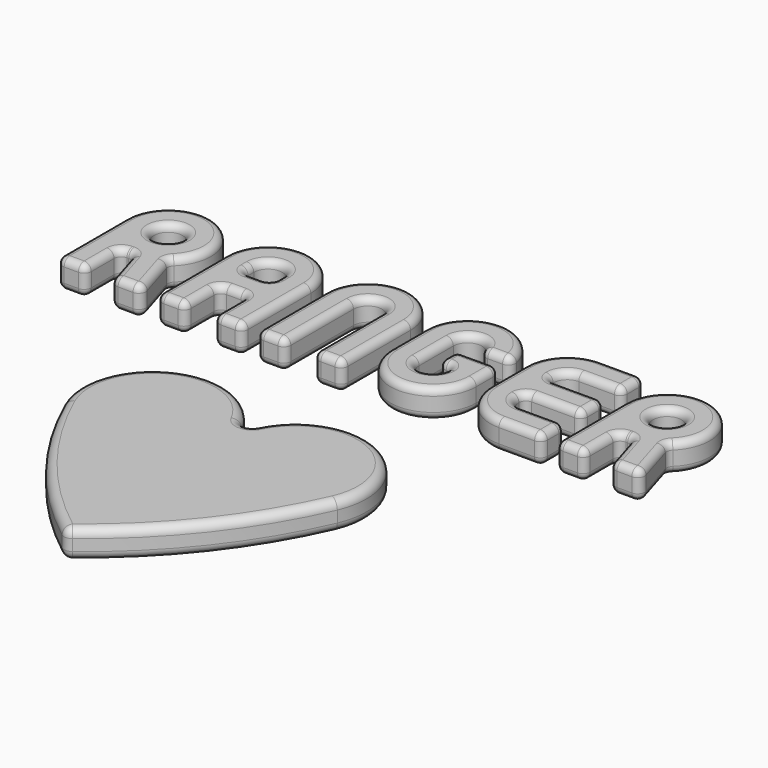
from build123d import *

# Parameters (mm, degrees)
F1_DEPTH = 1
F0_R     = 0.5
F2_R     = 0.24999
F2_2_R   = 0.24999
F2_3_R   = 0.24999
F2_4_R   = 0.24999
F2_5_R   = 0.24999
F2_6_R   = 0.24999
F4_DEPTH = 1
F5_R     = 0.3


# Not quite as in the source:
# - a fillet or chamfer is up to 0.001 mm smaller than in the source, because OpenCascade refuses the exact size


with BuildPart() as f1:
    # F0 (on Top) → F1 (new body)
    with BuildSketch(Plane.XY):
        with BuildLine():
            ThreePointArc((-12, 3), (-13.5, 4.5), (-15, 3))
            Line((-15, 3), (-15, 0))
            Line((-15, 0), (-14, 0))
            Line((-14, 0), (-14, 1.5))
            Line((-14, 1.5), (-13, 1.5))
            Line((-13, 1.5), (-13, 0))
            Line((-13, 0), (-12, 0))
            Line((-12, 0), (-12, 3))
        make_face()
        with BuildLine():
            ThreePointArc((-14, 3), (-13.5, 3.5), (-13, 3))
            Line((-13, 3), (-13, 2.5))
            Line((-13, 2.5), (-14, 2.5))
            Line((-14, 2.5), (-14, 3))
        make_face(mode=Mode.SUBTRACT)
    extrude(amount=F1_DEPTH)

    # F2#2 (radius 0.25 in the source; OpenCascade refuses exactly that, so slightly less here)
    f2_2_edges = [f1.edges().sort_by_distance(p)[0] for p in [
        (-13.5, 4.5, 1),
        (-15, 1.5, 1),
        (-14.5, 0, 1),
        (-14, 0.75, 1),
        (-13.5, 1.5, 1),
        (-13, 0.75, 1),
        (-12.5, 0, 1),
        (-12, 1.5, 1),
        (-13.5, 3.5, 1),
        (-13, 2.75, 1),
        (-13.5, 2.5, 1),
        (-14, 2.75, 1),
        (-13.5, 4.5, 0),
        (-15, 1.5, 0),
        (-14.5, 0, 0),
        (-14, 0.75, 0),
        (-13.5, 1.5, 0),
        (-13, 0.75, 0),
        (-12.5, 0, 0),
        (-12, 1.5, 0),
        (-13.5, 3.5, 0),
        (-13, 2.75, 0),
        (-13.5, 2.5, 0),
        (-14, 2.75, 0),
        (-13, 0, 0.5),
        (-12, 0, 0.5),
        (-13, 2.5, 0.5),
        (-14, 2.5, 0.5),
        (-14, 1.5, 0.5),
        (-13, 1.5, 0.5),
        (-15, 0, 0.5),
        (-14, 0, 0.5),
    ]]
    fillet(f2_2_edges, radius=F2_2_R)


with BuildPart() as f1b:
    # F0 (on Top) → F1, piece 2 (new body)
    with BuildSketch(Plane.XY):
        with BuildLine():
            ThreePointArc((-8.5, 3), (-10, 4.5), (-11.5, 3))
            Line((-11.5, 3), (-11.5, 0))
            Line((-11.5, 0), (-10.5, 0))
            Line((-10.5, 0), (-10.5, 3))
            ThreePointArc((-10.5, 3), (-10, 3.5), (-9.5, 3))
            Line((-9.5, 3), (-9.5, 0))
            Line((-9.5, 0), (-8.5, 0))
            Line((-8.5, 0), (-8.5, 3))
        make_face()
    extrude(amount=F1_DEPTH)

    # F2#3 (radius 0.25 in the source; OpenCascade refuses exactly that, so slightly less here)
    f2_3_edges = [f1b.edges().sort_by_distance(p)[0] for p in [
        (-10, 4.5, 1),
        (-11.5, 1.5, 1),
        (-11, 0, 1),
        (-10.5, 1.5, 1),
        (-10, 3.5, 1),
        (-9.5, 1.5, 1),
        (-9, 0, 1),
        (-8.5, 1.5, 1),
        (-10, 4.5, 0),
        (-11.5, 1.5, 0),
        (-11, 0, 0),
        (-10.5, 1.5, 0),
        (-10, 3.5, 0),
        (-9.5, 1.5, 0),
        (-9, 0, 0),
        (-8.5, 1.5, 0),
        (-9.5, 0, 0.5),
        (-8.5, 0, 0.5),
        (-11.5, 0, 0.5),
        (-10.5, 0, 0.5),
    ]]
    fillet(f2_3_edges, radius=F2_3_R)


with BuildPart() as f1c:
    # F0 (on Top) → F1, piece 3 (new body)
    with BuildSketch(Plane.XY):
        with BuildLine():
            Line((-7, 1.5), (-7, 3))
            ThreePointArc((-7, 3), (-6.5, 3.5), (-6, 3))
            Line((-6, 3), (-5, 3))
            ThreePointArc((-5, 3), (-6.5, 4.5), (-8, 3))
            Line((-8, 3), (-8, 1.5))
            ThreePointArc((-8, 1.5), (-6.5, 0), (-5, 1.5))
            Line((-5, 1.5), (-5, 2.5))
            Line((-5, 2.5), (-6.5, 2.5))
            Line((-6.5, 2.5), (-6.5, 1.75))
            Line((-6.5, 1.75), (-6, 1.75))
            Line((-6, 1.75), (-6, 1.5))
            ThreePointArc((-6, 1.5), (-6.5, 1), (-7, 1.5))
        make_face()
    extrude(amount=F1_DEPTH)

    # F2#4 (radius 0.25 in the source; OpenCascade refuses exactly that, so slightly less here)
    f2_4_edges = [f1c.edges().sort_by_distance(p)[0] for p in [
        (-6, 1.625, 1),
        (-6.5, 1, 1),
        (-7, 2.25, 1),
        (-6.5, 3.5, 1),
        (-5.5, 3, 1),
        (-6.5, 4.5, 1),
        (-8, 2.25, 1),
        (-6.5, 0, 1),
        (-5, 2, 1),
        (-5.75, 2.5, 1),
        (-6.5, 2.125, 1),
        (-6.25, 1.75, 1),
        (-6, 1.625, 0),
        (-6.5, 1, 0),
        (-7, 2.25, 0),
        (-6.5, 3.5, 0),
        (-5.5, 3, 0),
        (-6.5, 4.5, 0),
        (-8, 2.25, 0),
        (-6.5, 0, 0),
        (-5, 2, 0),
        (-5.75, 2.5, 0),
        (-6.5, 2.125, 0),
        (-6.25, 1.75, 0),
        (-5, 2.5, 0.5),
        (-6.5, 2.5, 0.5),
        (-6, 1.5, 0.5),
        (-7, 1.5, 0.5),
        (-8, 1.5, 0.5),
        (-5, 1.5, 0.5),
        (-6.5, 1.75, 0.5),
        (-6, 1.75, 0.5),
        (-6, 3, 0.5),
        (-5, 3, 0.5),
        (-7, 3, 0.5),
    ]]
    fillet(f2_4_edges, radius=F2_4_R)


with BuildPart() as f1d:
    # F0 (on Top) → F1, piece 4 (new body)
    with BuildSketch(Plane.XY):
        with BuildLine():
            ThreePointArc((-3, 4.5), (-4.0606601718, 4.0606601718), (-4.5, 3))
            Line((-4.5, 3), (-4.5, 1.5))
            ThreePointArc((-4.5, 1.5), (-4.0606601718, 0.4393398282), (-3, 0))
            Line((-3, 0), (-1.5, 0))
            Line((-1.5, 0), (-1.5, 1))
            Line((-1.5, 1), (-3, 1))
            ThreePointArc((-3, 1), (-3.3535533906, 1.1464466094), (-3.5, 1.5))
            Line((-3.5, 1.5), (-3.5, 1.75))
            Line((-3.5, 1.75), (-1.5, 1.75))
            Line((-1.5, 1.75), (-1.5, 2.75))
            Line((-1.5, 2.75), (-3.5, 2.75))
            Line((-3.5, 2.75), (-3.5, 3))
            ThreePointArc((-3.5, 3), (-3.3535533906, 3.3535533906), (-3, 3.5))
            Line((-3, 3.5), (-1.5, 3.5))
            Line((-1.5, 3.5), (-1.5, 4.5))
            Line((-1.5, 4.5), (-3, 4.5))
        make_face()
    extrude(amount=F1_DEPTH)

    # F2#5 (radius 0.25 in the source; OpenCascade refuses exactly that, so slightly less here)
    f2_5_edges = [f1d.edges().sort_by_distance(p)[0] for p in [
        (-4.06066, 4.06066, 1),
        (-4.5, 2.25, 1),
        (-4.06066, 0.43934, 1),
        (-2.25, 0, 1),
        (-1.5, 0.5, 1),
        (-2.25, 1, 1),
        (-3.353553, 1.146447, 1),
        (-3.5, 1.625, 1),
        (-2.5, 1.75, 1),
        (-1.5, 2.25, 1),
        (-2.5, 2.75, 1),
        (-3.5, 2.875, 1),
        (-3.353553, 3.353553, 1),
        (-2.25, 3.5, 1),
        (-1.5, 4, 1),
        (-2.25, 4.5, 1),
        (-4.06066, 4.06066, 0),
        (-4.5, 2.25, 0),
        (-4.06066, 0.43934, 0),
        (-2.25, 0, 0),
        (-1.5, 0.5, 0),
        (-2.25, 1, 0),
        (-3.353553, 1.146447, 0),
        (-3.5, 1.625, 0),
        (-2.5, 1.75, 0),
        (-1.5, 2.25, 0),
        (-2.5, 2.75, 0),
        (-3.5, 2.875, 0),
        (-3.353553, 3.353553, 0),
        (-2.25, 3.5, 0),
        (-1.5, 4, 0),
        (-2.25, 4.5, 0),
        (-3, 0, 0.5),
        (-1.5, 0, 0.5),
        (-1.5, 1, 0.5),
        (-3.5, 1.75, 0.5),
        (-1.5, 1.75, 0.5),
        (-3, 1, 0.5),
        (-1.5, 2.75, 0.5),
        (-3.5, 2.75, 0.5),
        (-3, 3.5, 0.5),
        (-1.5, 3.5, 0.5),
        (-1.5, 4.5, 0.5),
        (-3, 4.5, 0.5),
    ]]
    fillet(f2_5_edges, radius=F2_5_R)


with BuildPart() as f1e:
    # F0 (on Top) → F1, piece 5 (new body)
    with BuildSketch(Plane.XY):
        with BuildLine():
            Line((-1, 3), (-1, 0))
            Line((-1, 0), (0, 0))
            Line((0, 0), (0, 1.5))
            Line((0, 1.5), (0.5, 1.5))
            Line((0.5, 1.5), (0.9550055679, 0))
            Line((0.9550055679, 0), (2, 0))
            Line((2, 0), (1.4436707022, 1.8340301866))
            ThreePointArc((1.4436707022, 1.8340301866), (1.1459465716, 4.3537920914), (-1, 3))
        make_face()
        with Locations((0.5, 3)):
            Circle(F0_R, mode=Mode.SUBTRACT)
    extrude(amount=F1_DEPTH)

    # F2#6 (radius 0.25 in the source; OpenCascade refuses exactly that, so slightly less here)
    f2_6_edges = [f1e.edges().sort_by_distance(p)[0] for p in [
        (1.145947, 4.353792, 1),
        (-1, 1.5, 1),
        (-0.5, 0, 1),
        (0, 0.75, 1),
        (0.25, 1.5, 1),
        (0.727503, 0.75, 1),
        (1.477503, 0, 1),
        (1.721835, 0.917015, 1),
        (0, 3, 1),
        (1.145947, 4.353792, 0),
        (-1, 1.5, 0),
        (-0.5, 0, 0),
        (0, 0.75, 0),
        (0.25, 1.5, 0),
        (0.727503, 0.75, 0),
        (1.477503, 0, 0),
        (1.721835, 0.917015, 0),
        (0, 3, 0),
        (0.955006, 0, 0.5),
        (2, 0, 0.5),
        (-1, 0, 0.5),
        (0, 0, 0.5),
        (0, 1.5, 0.5),
        (0.5, 1.5, 0.5),
        (1.443671, 1.83403, 0.5),
        (-1, 3, 0.5),
    ]]
    fillet(f2_6_edges, radius=F2_6_R)


with BuildPart() as f1f:
    # F0 (on Top) → F1, piece 6 (new body)
    with BuildSketch(Plane.XY):
        with BuildLine():
            Line((-18.5, 3), (-18.5, 0))
            Line((-18.5, 0), (-17.5, 0))
            Line((-17.5, 0), (-17.5, 1.5))
            Line((-17.5, 1.5), (-17, 1.5))
            Line((-17, 1.5), (-16.5449944321, 0))
            Line((-16.5449944321, 0), (-15.5, 0))
            Line((-15.5, 0), (-16.0563292978, 1.8340301866))
            ThreePointArc((-16.0563292978, 1.8340301866), (-16.3540534284, 4.3537920914), (-18.5, 3))
        make_face()
        with Locations((-17, 3)):
            Circle(F0_R, mode=Mode.SUBTRACT)
    extrude(amount=F1_DEPTH)

    # F2 (radius 0.25 in the source; OpenCascade refuses exactly that, so slightly less here)
    f2_edges = [f1f.edges().sort_by_distance(p)[0] for p in [
        (-16.354053, 4.353792, 1),
        (-18.5, 1.5, 1),
        (-18, 0, 1),
        (-17.5, 0.75, 1),
        (-17.25, 1.5, 1),
        (-16.772497, 0.75, 1),
        (-16.022497, 0, 1),
        (-15.778165, 0.917015, 1),
        (-17.5, 3, 1),
        (-16.354053, 4.353792, 0),
        (-18.5, 1.5, 0),
        (-18, 0, 0),
        (-17.5, 0.75, 0),
        (-17.25, 1.5, 0),
        (-16.772497, 0.75, 0),
        (-16.022497, 0, 0),
        (-15.778165, 0.917015, 0),
        (-17.5, 3, 0),
        (-16.544994, 0, 0.5),
        (-15.5, 0, 0.5),
        (-18.5, 0, 0.5),
        (-17.5, 0, 0.5),
        (-17.5, 1.5, 0.5),
        (-17, 1.5, 0.5),
        (-16.056329, 1.83403, 0.5),
    ]]
    fillet(f2_edges, radius=F2_R)


with BuildPart() as f4:
    # F3 (on Top) → F4 (new body)
    with BuildSketch(Plane.XY):
        with BuildLine():
            ThreePointArc((-3.4629523531, -6.5096598739), (-5.2340635297, -3.0538173497), (-8.25, -5.5))
            ThreePointArc((-8.25, -5.5), (-11.2659364703, -3.0538173497), (-13.0370476469, -6.5096598739))
            ThreePointArc((-13.0370476469, -6.5096598739), (-11.0327775306, -9.8158934165), (-8.25, -12.5))
            ThreePointArc((-8.25, -12.5), (-5.4672224694, -9.8158934165), (-3.4629523531, -6.5096598739))
        make_face()
    extrude(amount=F4_DEPTH)

    # F5
    f5_edges = [f4.edges().sort_by_distance(p)[0] for p in [
        (-8.25, -5.5, 0.5),
        (-13.037048, -6.50966, 0.5),
        (-11.265936, -3.053817, 0),
        (-11.265936, -3.053817, 1),
        (-3.462952, -6.50966, 0.5),
        (-5.234064, -3.053817, 0),
        (-5.234064, -3.053817, 1),
        (-8.25, -12.5, 0.5),
    ]]
    fillet(f5_edges, radius=F5_R)


solid = Compound([f1.part, f1b.part, f1c.part, f1d.part, f1e.part, f1f.part, f4.part])
